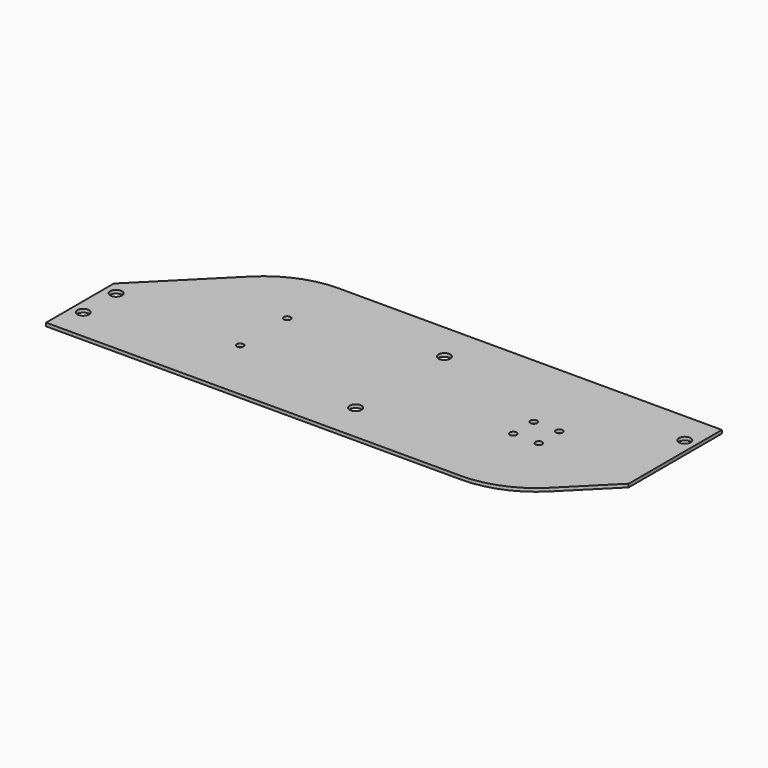
from build123d import *

# Parameters (mm, degrees)
F0_R     = 3.175
F0_R_2   = 1.8288
F1_DEPTH = 1.778


with BuildPart() as f1:
    # F0 (on Top) → F1 (new body)
    with BuildSketch(Plane.XY):
        with BuildLine():
            Line((133.35, -12.1520489686), (133.35, 50.8))
            Line((133.35, 50.8), (73.66, 50.8))
            ThreePointArc((73.66, 50.8), (109.5810244843, 35.9210244843), (124.46, 0))
            ThreePointArc((124.46, 0), (120.5930802516, -19.4403183641), (109.5810244843, -35.9210244843))
            Line((109.5810244843, -35.9210244843), (133.35, -12.1520489686))
        make_face()
        with Locations((127, 33.655)):
            Circle(F0_R, mode=Mode.SUBTRACT)
        with BuildLine():
            ThreePointArc((73.66, -50.8), (22.86, 0), (73.66, 50.8))
            Line((73.66, 50.8), (-73.6599997452, 50.8))
            ThreePointArc((-73.6599997452, 50.8), (-37.7389754256, 35.9210243942), (-22.86, 0))
            ThreePointArc((-22.86, 0), (-37.7389756058, -35.9210245744), (-73.6600002548, -50.8))
            Line((-73.6600002548, -50.8), (73.66, -50.8))
        make_face()
        with Locations((0, -29.972)):
            Circle(F0_R, mode=Mode.SUBTRACT)
        with Locations((0, 29.972)):
            Circle(F0_R, mode=Mode.SUBTRACT)
        with BuildLine():
            ThreePointArc((124.46, 0), (109.5810244843, 35.9210244843), (73.66, 50.8))
            ThreePointArc((73.66, 50.8), (22.86, 0), (73.66, -50.8))
            ThreePointArc((73.66, -50.8), (93.1003183641, -46.9330802516), (109.5810244843, -35.9210244843))
            ThreePointArc((109.5810244843, -35.9210244843), (120.5930802516, -19.4403183641), (124.46, 0))
        make_face()
        with Locations((66.7452027868, -6.9147972132)):
            Circle(F0_R_2, mode=Mode.SUBTRACT)
        with Locations((80.5747972132, -6.9147972132)):
            Circle(F0_R_2, mode=Mode.SUBTRACT)
        with Locations((66.7452027868, 6.9147972132)):
            Circle(F0_R_2, mode=Mode.SUBTRACT)
        with Locations((80.5747972132, 6.9147972132)):
            Circle(F0_R_2, mode=Mode.SUBTRACT)
        with BuildLine():
            ThreePointArc((-22.86, 0), (-37.7389754256, 35.9210243942), (-73.6599997452, 50.8))
            ThreePointArc((-73.6599997452, 50.8), (-93.1003182465, 46.9330803003), (-109.5810244843, 35.9210244843))
            ThreePointArc((-109.5810244843, 35.9210244843), (-120.5930803003, -19.4403182465), (-73.6600002548, -50.8))
            ThreePointArc((-73.6600002548, -50.8), (-37.7389756058, -35.9210245744), (-22.86, 0))
        make_face()
        with Locations((-73.66, -15.875)):
            Circle(F0_R_2, mode=Mode.SUBTRACT)
        with Locations((-73.66, 15.875)):
            Circle(F0_R_2, mode=Mode.SUBTRACT)
        with BuildLine():
            ThreePointArc((-73.6600002548, -50.8), (-120.5930803003, -19.4403182465), (-109.5810244843, 35.9210244843))
            Line((-109.5810244843, 35.9210244843), (-133.35, 12.1520489686))
            Line((-133.35, 12.1520489686), (-133.35, -50.8))
            Line((-133.35, -50.8), (-73.6600002548, -50.8))
        make_face()
        Polygon((-133.35, -50.8), (-133.35, 12.1520489686), (-150.5712, -5.0691510314), (-150.5712, -50.8), align=None)
        with Locations((-144.2212, -33.655)):
            Circle(F0_R, mode=Mode.SUBTRACT)
        with Locations((-144.2212, -11.43)):
            Circle(F0_R, mode=Mode.SUBTRACT)
    extrude(amount=F1_DEPTH)


solid = f1.part
